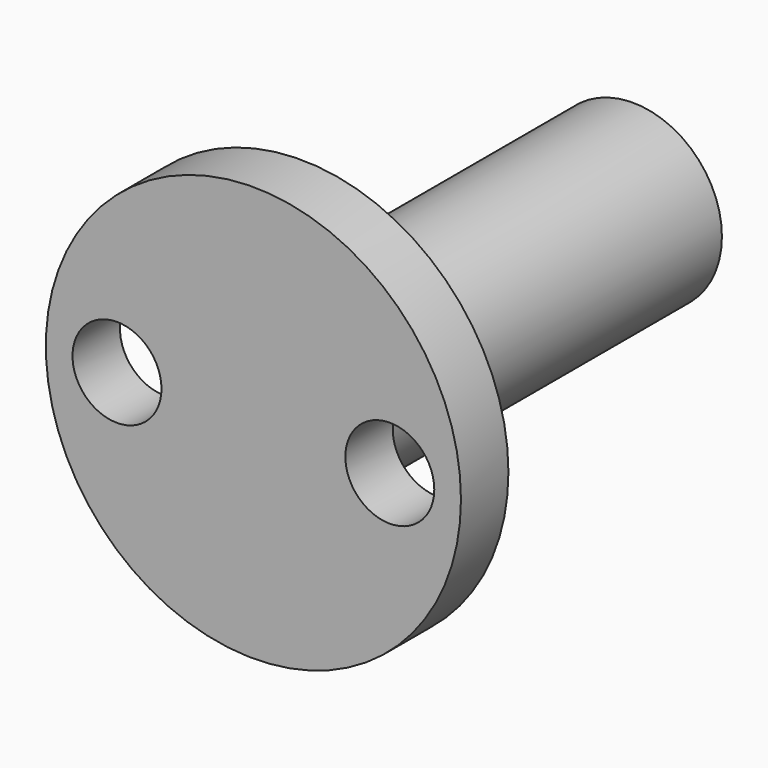
from build123d import *

# Parameters (mm, degrees)
F0_R     = 7
F0_R_2   = 1.5
F0_R_3   = 3
F1_DEPTH = 2
F2_DEPTH = 14
F3_R     = 2.05
F4_DEPTH = 14


# Not quite as in the source:
# - a feature names something its author has since deleted; it is built from what else it names


with BuildPart() as f1:
    # F0 (on Front) → F1 (new body)
    with BuildSketch(Plane.XZ):
        Circle(F0_R)
        with Locations((-4.6, 0)):
            Circle(F0_R_2, mode=Mode.SUBTRACT)
        Circle(F0_R_3, mode=Mode.SUBTRACT)
        with Locations((4.6, 0)):
            Circle(F0_R_2, mode=Mode.SUBTRACT)
        Circle(F0_R_3)
    extrude(amount=F1_DEPTH)

    # F0 (on Front) → F2 (join)
    with BuildSketch(Plane.XZ):
        Circle(F0_R_3)
    extrude(amount=-F2_DEPTH)

    # F3 (on face) → F4 (cut)
    with BuildSketch(Plane(origin=(0, 14, 0), x_dir=(-1, 0, 0), z_dir=(0, 1, 0))):
        Circle(F3_R)
    extrude(amount=-F4_DEPTH, mode=Mode.SUBTRACT)


solid = f1.part
